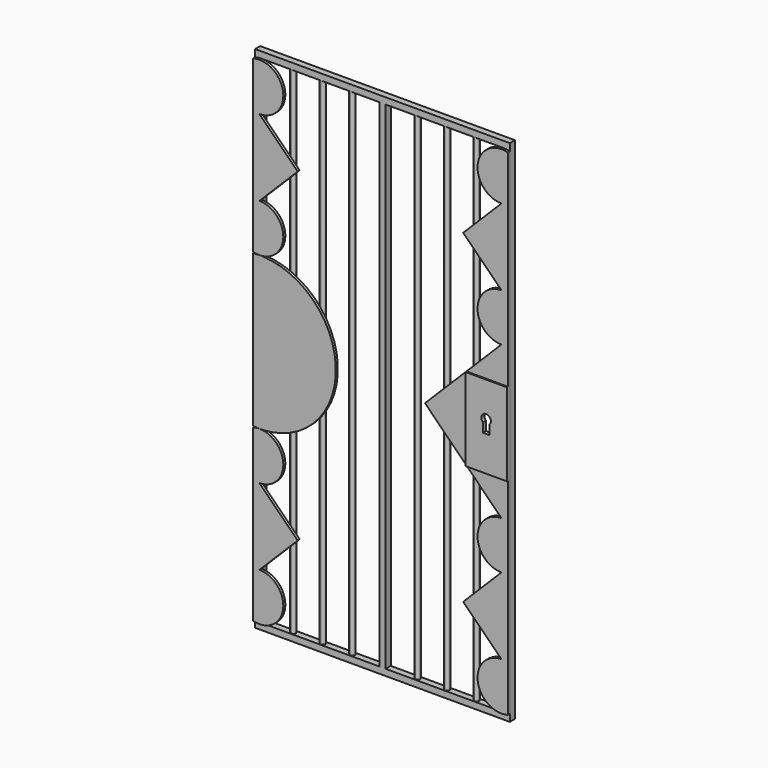
from build123d import *

# Parameters (mm, degrees)
F0_W      = 25
F0_H      = 25
F0_H_2    = 1950
F0_W_2    = 950
F1_DEPTH  = 25
F3_DEPTH  = 1975
F5_DEPTH  = 10
F7_DEPTH  = 1975
F9_DEPTH  = 1975
F10_W     = 162.5
F10_H     = 325
F11_DEPTH = 5
F13_DEPTH = 86.3


# Not quite as in the source:
# - ends of sketch curves that miss each other by under 0.0002 mm in the source are joined


with BuildPart() as f1:
    # F0 (on Front) → F1 (new body)
    with BuildSketch(Plane.XZ):
        with Locations((487.5, 0)):
            Rectangle(F0_W, F0_H)
        with Locations((487.5, 987.5)):
            Rectangle(F0_W, F0_H_2)
        Rectangle(F0_W_2, F0_H)
        with Locations((487.5, 1975)):
            Rectangle(F0_W, F0_H)
        with Locations((-487.5, 0)):
            Rectangle(F0_W, F0_H)
        with Locations((-487.5, 987.5)):
            Rectangle(F0_W, F0_H_2)
        with Locations((0, 1975)):
            Rectangle(F0_W_2, F0_H)
        with Locations((-487.5, 1975)):
            Rectangle(F0_W, F0_H)
    extrude(amount=F1_DEPTH)

    # F2 (on Top) → F3 (join)
    with BuildSketch(Plane.XY):
        Polygon((12.5, 0), (0, 0), (-12.5, 0), (-12.5, -25), (0, -25), (12.5, -25), align=None)
    extrude(amount=F3_DEPTH)

    # F6 (on face) → F7 (join)
    with BuildSketch(Plane(origin=(0, 0, 1962.5), x_dir=(1, 0, 0), z_dir=(0, 0, -1))):
        with BuildLine():
            Line((-128.125, 2.5), (-128.125, 22.5))
            ThreePointArc((-128.125, 22.5), (-138.125, 12.5), (-128.125, 2.5))
        make_face()
        with BuildLine():
            ThreePointArc((-118.125, 12.5), (-121.0539321881, 19.5710678119), (-128.125, 22.5))
            Line((-128.125, 22.5), (-128.125, 2.5))
            ThreePointArc((-128.125, 2.5), (-121.0539321881, 5.4289321881), (-118.125, 12.5))
        make_face()
        with BuildLine():
            Line((-359.375, 2.5), (-359.375, 22.5))
            ThreePointArc((-359.375, 22.5), (-369.375, 12.5), (-359.375, 2.5))
        make_face()
        with BuildLine():
            ThreePointArc((-349.375, 12.5), (-352.3039321881, 19.5710678119), (-359.375, 22.5))
            Line((-359.375, 22.5), (-359.375, 2.5))
            ThreePointArc((-359.375, 2.5), (-352.3039321881, 5.4289321881), (-349.375, 12.5))
        make_face()
        with BuildLine():
            ThreePointArc((-233.75, 12.5), (-236.6789321881, 19.5710678119), (-243.75, 22.5))
            Line((-243.75, 22.5), (-243.75, 2.5))
            ThreePointArc((-243.75, 2.5), (-236.6789321881, 5.4289321881), (-233.75, 12.5))
        make_face()
        with BuildLine():
            Line((-243.75, 2.5), (-243.75, 22.5))
            ThreePointArc((-243.75, 22.5), (-253.75, 12.5), (-243.75, 2.5))
        make_face()
    extrude(amount=F7_DEPTH)

    # F8 (on face) → F9 (join)
    with BuildSketch(Plane(origin=(0, 0, 1962.5), x_dir=(1, 0, 0), z_dir=(0, 0, -1))):
        with BuildLine():
            Line((128.125, 2.5), (128.125, 22.5))
            ThreePointArc((128.125, 22.5), (118.125, 12.5), (128.125, 2.5))
        make_face()
        with BuildLine():
            ThreePointArc((138.125, 12.5), (135.1960678119, 19.5710678119), (128.125, 22.5))
            Line((128.125, 22.5), (128.125, 2.5))
            ThreePointArc((128.125, 2.5), (135.1960678119, 5.4289321881), (138.125, 12.5))
        make_face()
        with BuildLine():
            Line((359.375, 2.5), (359.375, 22.5))
            ThreePointArc((359.375, 22.5), (349.375, 12.5), (359.375, 2.5))
        make_face()
        with BuildLine():
            ThreePointArc((369.375, 12.5), (366.4460678119, 19.5710678119), (359.375, 22.5))
            Line((359.375, 22.5), (359.375, 2.5))
            ThreePointArc((359.375, 2.5), (366.4460678119, 5.4289321881), (369.375, 12.5))
        make_face()
        with BuildLine():
            Line((243.75, 2.5), (243.75, 22.5))
            ThreePointArc((243.75, 22.5), (233.75, 12.5), (243.75, 2.5))
        make_face()
        with BuildLine():
            ThreePointArc((253.75, 12.5), (250.8210678119, 19.5710678119), (243.75, 22.5))
            Line((243.75, 22.5), (243.75, 2.5))
            ThreePointArc((243.75, 2.5), (250.8210678119, 5.4289321881), (253.75, 12.5))
        make_face()
    extrude(amount=F9_DEPTH)


with BuildPart() as f5:
    # F4 (on face) → F5 (new body)
    with BuildSketch(Plane.XZ.offset(25)):
        with BuildLine():
            ThreePointArc((500, 684.1052018425), (487.6147201171, 686.6474237337), (475, 687.5))
            Line((475, 687.5), (500, 662.5))
            Line((500, 662.5), (500, 684.1052018425))
        make_face()
        with BuildLine():
            Line((475, 500), (475, 687.5))
            ThreePointArc((475, 687.5), (381.25, 593.75), (475, 500))
        make_face()
        with BuildLine():
            Line((475, 1287.5), (475, 687.5))
            ThreePointArc((475, 687.5), (487.6147201171, 686.6474237337), (500, 684.1052018425))
            Line((500, 684.1052018425), (500, 1290.8947981575))
            ThreePointArc((500, 1290.8947981575), (487.6147201171, 1288.3525762663), (475, 1287.5))
        make_face()
        Polygon((175, 987.5), (475, 687.5), (475, 1287.5), align=None)
        Polygon((500, 662.5), (475, 687.5), (475, 500), (500, 525), align=None)
        with BuildLine():
            ThreePointArc((500, 503.3947981575), (487.6147201171, 500.8525762663), (475, 500))
            Line((475, 500), (475, 350))
            Line((475, 350), (475, 200))
            ThreePointArc((475, 200), (487.6147201171, 199.1474237337), (500, 196.6052018425))
            Line((500, 196.6052018425), (500, 503.3947981575))
        make_face()
        Polygon((475, 350), (475, 500), (325, 350), align=None)
        with BuildLine():
            Line((500, 525), (475, 500))
            ThreePointArc((475, 500), (487.6147201171, 500.8525762663), (500, 503.3947981575))
            Line((500, 503.3947981575), (500, 525))
        make_face()
        Polygon((475, 1475), (475, 1287.5), (500, 1312.5), (500, 1450), align=None)
        with BuildLine():
            Line((500, 1312.5), (475, 1287.5))
            ThreePointArc((475, 1287.5), (487.6147201171, 1288.3525762663), (500, 1290.8947981575))
            Line((500, 1290.8947981575), (500, 1312.5))
        make_face()
        with BuildLine():
            ThreePointArc((475, 1475), (381.25, 1381.25), (475, 1287.5))
            Line((475, 1287.5), (475, 1475))
        make_face()
        Polygon((475, 200), (475, 350), (325, 350), align=None)
        Polygon((325, 1625), (475, 1475), (475, 1625), align=None)
        with BuildLine():
            ThreePointArc((500, 1471.6052018425), (487.6147201171, 1474.1474237337), (475, 1475))
            Line((475, 1475), (500, 1450))
            Line((500, 1450), (500, 1471.6052018425))
        make_face()
        with BuildLine():
            Line((475, 1625), (475, 1475))
            ThreePointArc((475, 1475), (487.6147201171, 1474.1474237337), (500, 1471.6052018425))
            Line((500, 1471.6052018425), (500, 1778.3947981575))
            ThreePointArc((500, 1778.3947981575), (487.6147201171, 1775.8525762663), (475, 1775))
            Line((475, 1775), (475, 1625))
        make_face()
        with BuildLine():
            ThreePointArc((500, 196.6052018425), (487.6147201171, 199.1474237337), (475, 200))
            Line((475, 200), (500, 175))
            Line((500, 175), (500, 196.6052018425))
        make_face()
        with BuildLine():
            Line((475, 12.5), (475, 200))
            ThreePointArc((475, 200), (381.25, 106.25), (475, 12.5))
        make_face()
        with BuildLine():
            Line((500, 175), (475, 200))
            Line((475, 200), (475, 12.5))
            ThreePointArc((475, 12.5), (487.6147201171, 13.3525762663), (500, 15.8947981575))
            Line((500, 15.8947981575), (500, 175))
        make_face()
        Polygon((325, 1625), (475, 1625), (475, 1775), align=None)
        with BuildLine():
            Line((475, 1962.5), (475, 1775))
            Line((475, 1775), (500, 1800))
            Line((500, 1800), (500, 1959.1052018425))
            ThreePointArc((500, 1959.1052018425), (487.6147201171, 1961.6474237337), (475, 1962.5))
        make_face()
        with BuildLine():
            Line((500, 1800), (475, 1775))
            ThreePointArc((475, 1775), (487.6147201171, 1775.8525762663), (500, 1778.3947981575))
            Line((500, 1778.3947981575), (500, 1800))
        make_face()
        with BuildLine():
            ThreePointArc((475, 1962.5), (381.25, 1868.75), (475, 1775))
            Line((475, 1775), (475, 1962.5))
        make_face()
    extrude(amount=F5_DEPTH)

    # F10 (on face) → F11 (join)
    with BuildSketch(Plane.XZ.offset(35)):
        with Locations((418.75, 987.5)):
            Rectangle(F10_W, F10_H)
    extrude(amount=F11_DEPTH)

    # F12 (on face) → F13 (cut)
    with BuildSketch(Plane.XZ.offset(40)):
        with BuildLine():
            Line((406.25, 962.5), (431.25, 962.5))
            Line((431.25, 962.5), (431.25, 998.5245751406))
            ThreePointArc((431.25, 998.5245751406), (418.75, 993.75), (406.25, 998.5245751406))
            Line((406.25, 998.5245751406), (406.25, 962.5))
        make_face()
        with BuildLine():
            ThreePointArc((406.25, 998.5245751406), (418.75, 993.75), (431.25, 998.5245751406))
            ThreePointArc((431.25, 998.5245751406), (435.866329922, 1004.8453445538), (437.5, 1012.5))
            ThreePointArc((437.5, 1012.5), (411.0953445538, 1029.616329922), (406.25, 998.5245751406))
        make_face()
    extrude(amount=-F13_DEPTH, mode=Mode.SUBTRACT)


with BuildPart() as f5b:
    # F4 (on face) → F5, piece 2 (new body)
    with BuildSketch(Plane.XZ.offset(25)):
        with BuildLine():
            Line((-500, 175), (-500, 15.8947981575))
            ThreePointArc((-500, 15.8947981575), (-487.6147201171, 13.3525762663), (-475, 12.5))
            Line((-475, 12.5), (-475, 200))
            Line((-475, 200), (-500, 175))
        make_face()
        with BuildLine():
            Line((-500, 503.3947981575), (-500, 196.6052018425))
            ThreePointArc((-500, 196.6052018425), (-487.6147201171, 199.1474237337), (-475, 200))
            Line((-475, 200), (-475, 350))
            Line((-475, 350), (-475, 500))
            ThreePointArc((-475, 500), (-487.6147201171, 500.8525762663), (-500, 503.3947981575))
        make_face()
        with BuildLine():
            ThreePointArc((-475, 200), (-487.6147201171, 199.1474237337), (-500, 196.6052018425))
            Line((-500, 196.6052018425), (-500, 175))
            Line((-500, 175), (-475, 200))
        make_face()
        with BuildLine():
            Line((-475, 200), (-475, 12.5))
            ThreePointArc((-475, 12.5), (-408.7087392638, 39.9587392638), (-381.25, 106.25))
            ThreePointArc((-381.25, 106.25), (-408.7087392638, 172.5412607362), (-475, 200))
        make_face()
        Polygon((-475, 350), (-475, 200), (-325, 350), align=None)
        with BuildLine():
            Line((-500, 525), (-500, 503.3947981575))
            ThreePointArc((-500, 503.3947981575), (-487.6147201171, 500.8525762663), (-475, 500))
            Line((-475, 500), (-500, 525))
        make_face()
        Polygon((-475, 500), (-475, 350), (-325, 350), align=None)
        with BuildLine():
            ThreePointArc((-475, 687.5), (-487.6147201171, 686.6474237337), (-500, 684.1052018425))
            Line((-500, 684.1052018425), (-500, 525))
            Line((-500, 525), (-475, 500))
            Line((-475, 500), (-475, 687.5))
        make_face()
        with BuildLine():
            Line((-475, 687.5), (-475, 500))
            ThreePointArc((-475, 500), (-408.7087392638, 527.4587392638), (-381.25, 593.75))
            ThreePointArc((-381.25, 593.75), (-408.7087392638, 660.0412607362), (-475, 687.5))
        make_face()
    extrude(amount=F5_DEPTH)


with BuildPart() as f5c:
    # F4 (on face) → F5, piece 3 (new body)
    with BuildSketch(Plane.XZ.offset(25)):
        with BuildLine():
            ThreePointArc((-475, 1962.5), (-487.6147201171, 1961.6474237337), (-500, 1959.1052018425))
            Line((-500, 1959.1052018425), (-500, 1800))
            Line((-500, 1800), (-475, 1775))
            Line((-475, 1775), (-475, 1962.5))
        make_face()
        with BuildLine():
            ThreePointArc((-381.25, 1868.75), (-408.7087392638, 1935.0412607362), (-475, 1962.5))
            Line((-475, 1962.5), (-475, 1775))
            ThreePointArc((-475, 1775), (-408.7087392638, 1802.4587392638), (-381.25, 1868.75))
        make_face()
        with BuildLine():
            Line((-500, 1800), (-500, 1778.3947981575))
            ThreePointArc((-500, 1778.3947981575), (-487.6147201171, 1775.8525762663), (-475, 1775))
            Line((-475, 1775), (-500, 1800))
        make_face()
        with BuildLine():
            ThreePointArc((-475, 1775), (-487.6147201171, 1775.8525762663), (-500, 1778.3947981575))
            Line((-500, 1778.3947981575), (-500, 1471.6052018425))
            ThreePointArc((-500, 1471.6052018425), (-487.6147201171, 1474.1474237337), (-475, 1475))
            Line((-475, 1475), (-475, 1625))
            Line((-475, 1625), (-475, 1775))
        make_face()
        Polygon((-325, 1625), (-475, 1775), (-475, 1625), align=None)
        with BuildLine():
            ThreePointArc((-475, 1475), (-487.6147201171, 1474.1474237337), (-500, 1471.6052018425))
            Line((-500, 1471.6052018425), (-500, 1450))
            Line((-500, 1450), (-475, 1475))
        make_face()
        Polygon((-325, 1625), (-475, 1625), (-475, 1475), align=None)
        with BuildLine():
            Line((-475, 1287.5), (-475, 1475))
            Line((-475, 1475), (-500, 1450))
            Line((-500, 1450), (-500, 1290.8947981575))
            ThreePointArc((-500, 1290.8947981575), (-487.6147202668, 1288.3525762866), (-475, 1287.5))
        make_face()
        with BuildLine():
            ThreePointArc((-381.25, 1381.25), (-408.7087392638, 1447.5412607362), (-475, 1475))
            Line((-475, 1475), (-475, 1287.5))
            ThreePointArc((-475, 1287.5), (-408.7087393706, 1314.9587391569), (-381.25, 1381.25))
        make_face()
    extrude(amount=F5_DEPTH)


with BuildPart() as f5d:
    # F4 (on face) → F5, piece 4 (new body)
    with BuildSketch(Plane.XZ.offset(25)):
        with BuildLine():
            Line((-475, 1287.5), (-475, 687.5))
            ThreePointArc((-475, 687.5), (-262.867965644, 775.367965644), (-175, 987.5))
            ThreePointArc((-175, 987.5), (-262.8679657509, 1199.6320344628), (-475, 1287.5))
        make_face()
        with BuildLine():
            ThreePointArc((-500, 688.5434814225), (-487.5108837965, 687.7609838766), (-475, 687.5))
            Line((-475, 687.5), (-475, 1287.5))
            ThreePointArc((-475, 1287.5), (-487.5108839475, 1287.2390161171), (-500, 1286.4565185775))
            Line((-500, 1286.4565185775), (-500, 688.5434814225))
        make_face()
    extrude(amount=F5_DEPTH)


solid = Compound([f1.part, f5.part, f5b.part, f5c.part, f5d.part])
